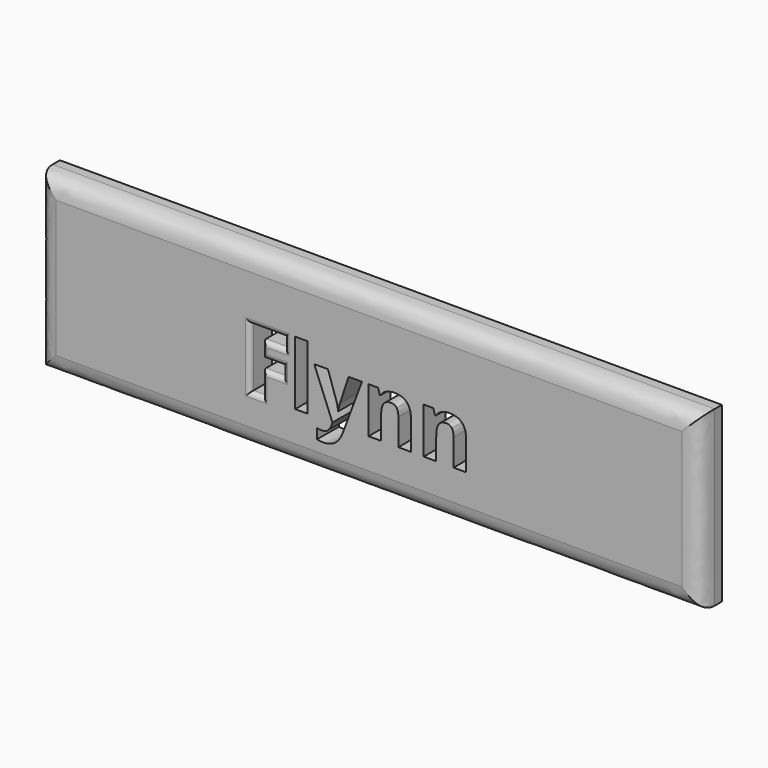
from build123d import *

# Parameters (mm, degrees)
F0_W        = 72.5492089987
F0_H        = 18.9791209996
F0_W_2      = 1.3700789067
F0_H_2      = 6.9912840748
F1_DEPTH    = 3
F2_T1_DEPTH = 82.5492089987
F2_T3_DEPTH = 28.9791209996
F3_R        = 0.5


# Not quite as in the source:
# - a fillet or chamfer that OpenCascade refuses, or shapes differently, is made with other operations: its cross-section is extruded or revolved along the edge and cut away or added


with BuildPart() as f1:
    # F0 (on Front) → F1 (new body)
    with BuildSketch(Plane.XZ):
        with Locations((-36.2746044993, 9.4895604998)):
            Rectangle(F0_W, F0_H)
        with BuildLine():
            Line((-40.2793404323, 5.3929338044), (-42.2747963845, 10.3801360367))
            Line((-42.2747963845, 10.3801360367), (-40.7738914752, 10.3801360367))
            Line((-40.7738914752, 10.3801360367), (-39.8264811924, 7.5537193204))
            add(Edge.make_bspline(
                [(-39.8264811924, 7.5537193204), (-39.70428108, 7.185681335), (-39.6597139803, 6.6825044018)],
                knots=[0, 0, 0, 1, 1, 1], degree=2))
            Line((-39.6597139803, 6.6825044018), (-39.632398661, 6.6825044018))
            add(Edge.make_bspline(
                [(-39.632398661, 6.6825044018), (-39.5835186161, 7.1454271804), (-39.439753778, 7.5537193204)],
                knots=[0, 0, 0, 1, 1, 1], degree=2))
            Line((-39.439753778, 7.5537193204), (-38.5095952758, 10.3801360367))
            Line((-38.5095952758, 10.3801360367), (-37.0403186308, 10.3801360367))
            Line((-37.0403186308, 10.3801360367), (-39.1651629373, 4.7143637688))
            add(Edge.make_bspline(
                [(-39.1651629373, 4.7143637688), (-39.458443207, 3.9279701046), (-39.9997178223, 3.5369297451)],
                knots=[0, 0, 0, 1, 1, 1], degree=2))
            add(Edge.make_bspline(
                [(-39.9997178223, 3.5369297451), (-40.5409924376, 3.1458893856), (-41.264129573, 3.1458893856)],
                knots=[0, 0, 0, 1, 1, 1], degree=2))
            add(Edge.make_bspline(
                [(-41.264129573, 3.1458893856), (-41.619228723, 3.1458893856), (-41.9599513892, 3.2235223981)],
                knots=[0, 0, 0, 1, 1, 1], degree=2))
            Line((-41.9599513892, 3.2235223981), (-41.9599513892, 4.3103845738))
            add(Edge.make_bspline(
                [(-41.9599513892, 4.3103845738), (-41.7126758677, 4.2514409902), (-41.4208332465, 4.2514409902)],
                knots=[0, 0, 0, 1, 1, 1], degree=2))
            add(Edge.make_bspline(
                [(-41.4208332465, 4.2514409902), (-41.0571082062, 4.2514409902), (-40.7853926623, 4.4742764892)],
                knots=[0, 0, 0, 1, 1, 1], degree=2))
            add(Edge.make_bspline(
                [(-40.7853926623, 4.4742764892), (-40.5136771183, 4.6971119882), (-40.36128639, 5.145658283)],
                knots=[0, 0, 0, 1, 1, 1], degree=2))
            Line((-40.36128639, 5.145658283), (-40.2793404323, 5.3929338044))
        make_face(mode=Mode.SUBTRACT)
        Polygon((-47.9362557073, 7.9533855702), (-47.9362557073, 5.3569925949), (-49.306334614, 5.3569925949), (-49.306334614, 11.9256080458), (-45.5411335052, 11.9256080458), (-45.5411335052, 10.7841152316), (-47.9362557073, 10.7841152316), (-47.9362557073, 9.0905654393), (-45.7079007174, 9.0905654393), (-45.7079007174, 7.9533855702), align=None, mode=Mode.SUBTRACT)
        with Locations((-43.6786600282, 8.8526346323)):
            Rectangle(F0_W_2, F0_H_2, mode=Mode.SUBTRACT)
        with BuildLine():
            Line((-31.6850784131, 8.6319556059), (-31.6850784131, 5.3569925949))
            Line((-31.6850784131, 5.3569925949), (-33.0551573198, 5.3569925949))
            Line((-33.0551573198, 5.3569925949), (-33.0551573198, 8.2912329397))
            add(Edge.make_bspline(
                [(-33.0551573198, 8.2912329397), (-33.0551573198, 8.8346640275), (-33.248521027, 9.1063795715)],
                knots=[0, 0, 0, 1, 1, 1], degree=2))
            add(Edge.make_bspline(
                [(-33.248521027, 9.1063795715), (-33.4418847342, 9.3780951154), (-33.8645533581, 9.3780951154)],
                knots=[0, 0, 0, 1, 1, 1], degree=2))
            add(Edge.make_bspline(
                [(-33.8645533581, 9.3780951154), (-34.4396127103, 9.3780951154), (-34.6955141221, 8.9942429978)],
                knots=[0, 0, 0, 1, 1, 1], degree=2))
            add(Edge.make_bspline(
                [(-34.6955141221, 8.9942429978), (-34.9514155338, 8.6103908802), (-34.9514155338, 7.7204865326)],
                knots=[0, 0, 0, 1, 1, 1], degree=2))
            Line((-34.9514155338, 7.7204865326), (-34.9514155338, 5.3569925949))
            Line((-34.9514155338, 5.3569925949), (-36.3214944405, 5.3569925949))
            Line((-36.3214944405, 5.3569925949), (-36.3214944405, 10.3801360367))
            Line((-36.3214944405, 10.3801360367), (-35.2748864195, 10.3801360367))
            Line((-35.2748864195, 10.3801360367), (-35.0908674267, 9.7375072106))
            Line((-35.0908674267, 9.7375072106), (-35.0146720626, 9.7375072106))
            add(Edge.make_bspline(
                [(-35.0146720626, 9.7375072106), (-34.7846483217, 10.1012322508), (-34.3828255993, 10.2874077161)],
                knots=[0, 0, 0, 1, 1, 1], degree=2))
            add(Edge.make_bspline(
                [(-34.3828255993, 10.2874077161), (-33.9810028769, 10.4735831814), (-33.4692000534, 10.4735831814)],
                knots=[0, 0, 0, 1, 1, 1], degree=2))
            add(Edge.make_bspline(
                [(-33.4692000534, 10.4735831814), (-32.5922345413, 10.4735831814), (-32.1386564772, 9.99987804)],
                knots=[0, 0, 0, 1, 1, 1], degree=2))
            add(Edge.make_bspline(
                [(-32.1386564772, 9.99987804), (-31.6850784131, 9.5261728986), (-31.6850784131, 8.6319556059)],
                knots=[0, 0, 0, 1, 1, 1], degree=2))
        make_face(mode=Mode.SUBTRACT)
        with BuildLine():
            Line((-25.6383293244, 8.6319556059), (-25.6383293244, 5.3569925949))
            Line((-25.6383293244, 5.3569925949), (-27.0084082311, 5.3569925949))
            Line((-27.0084082311, 5.3569925949), (-27.0084082311, 8.2912329397))
            add(Edge.make_bspline(
                [(-27.0084082311, 8.2912329397), (-27.0084082311, 8.8346640275), (-27.2017719383, 9.1063795715)],
                knots=[0, 0, 0, 1, 1, 1], degree=2))
            add(Edge.make_bspline(
                [(-27.2017719383, 9.1063795715), (-27.3951356454, 9.3780951154), (-27.8178042693, 9.3780951154)],
                knots=[0, 0, 0, 1, 1, 1], degree=2))
            add(Edge.make_bspline(
                [(-27.8178042693, 9.3780951154), (-28.3928636216, 9.3780951154), (-28.6487650333, 8.9942429978)],
                knots=[0, 0, 0, 1, 1, 1], degree=2))
            add(Edge.make_bspline(
                [(-28.6487650333, 8.9942429978), (-28.9046664451, 8.6103908802), (-28.9046664451, 7.7204865326)],
                knots=[0, 0, 0, 1, 1, 1], degree=2))
            Line((-28.9046664451, 7.7204865326), (-28.9046664451, 5.3569925949))
            Line((-28.9046664451, 5.3569925949), (-30.2747453518, 5.3569925949))
            Line((-30.2747453518, 5.3569925949), (-30.2747453518, 10.3801360367))
            Line((-30.2747453518, 10.3801360367), (-29.2281373307, 10.3801360367))
            Line((-29.2281373307, 10.3801360367), (-29.044118338, 9.7375072106))
            Line((-29.044118338, 9.7375072106), (-28.9679229738, 9.7375072106))
            add(Edge.make_bspline(
                [(-28.9679229738, 9.7375072106), (-28.7378992329, 10.1012322508), (-28.3360765105, 10.2874077161)],
                knots=[0, 0, 0, 1, 1, 1], degree=2))
            add(Edge.make_bspline(
                [(-28.3360765105, 10.2874077161), (-27.9342537882, 10.4735831814), (-27.4224509647, 10.4735831814)],
                knots=[0, 0, 0, 1, 1, 1], degree=2))
            add(Edge.make_bspline(
                [(-27.4224509647, 10.4735831814), (-26.5454854525, 10.4735831814), (-26.0919073884, 9.99987804)],
                knots=[0, 0, 0, 1, 1, 1], degree=2))
            add(Edge.make_bspline(
                [(-26.0919073884, 9.99987804), (-25.6383293244, 9.5261728986), (-25.6383293244, 8.6319556059)],
                knots=[0, 0, 0, 1, 1, 1], degree=2))
        make_face(mode=Mode.SUBTRACT)
    extrude(amount=F1_DEPTH)

    # F2: fillet of radius 2 on 4 edges, made by hand

    # F2_s2 → F2_t1 (cut)
    with BuildSketch(Plane.YZ.offset(-77.5492089987)):
        with BuildLine():
            add(Edge.make_bspline(
                [(-1, 18.9791209996), (-3, 18.9791209996), (-3, 16.9791209996)],
                knots=[0, 0, 0, 1, 1, 1], degree=2, weights=[1, 1, 1]))
            Line((-3, 16.9791209996), (-3, 18.9791209996))
            Line((-3, 18.9791209996), (-1, 18.9791209996))
        make_face()
        with BuildLine():
            add(Edge.make_bspline(
                [(-1, 0), (-3, 0), (-3, 2)],
                knots=[0, 0, 0, 1, 1, 1], degree=2, weights=[1, 1, 1]))
            Line((-3, 2), (-3, 0))
            Line((-3, 0), (-1, 0))
        make_face()
    extrude(amount=F2_T1_DEPTH, mode=Mode.SUBTRACT)

    # F2_s4 → F2_t3 (cut)
    with BuildSketch(Plane.XY.offset(-5)):
        with BuildLine():
            add(Edge.make_bspline(
                [(-72.5492089987, -1), (-72.5492089987, -3), (-70.5492089987, -3)],
                knots=[0, 0, 0, 1, 1, 1], degree=2, weights=[1, 1, 1]))
            Line((-70.5492089987, -3), (-72.5492089987, -3))
            Line((-72.5492089987, -3), (-72.5492089987, -1))
        make_face()
        with BuildLine():
            add(Edge.make_bspline(
                [(0, -1), (0, -3), (-2, -3)],
                knots=[0, 0, 0, 1, 1, 1], degree=2, weights=[1, 1, 1]))
            Line((-2, -3), (0, -3))
            Line((0, -3), (0, -1))
        make_face()
    extrude(amount=F2_T3_DEPTH, mode=Mode.SUBTRACT)

    # F3
    f3_edges = [f1.edges().sort_by_distance(p)[0] for p in [
        (-49.306335, -3, 8.6413),
        (-47.423734, -3, 11.925608),
        (-45.541134, -3, 11.354862),
        (-46.738695, -3, 10.784115),
        (-47.936256, -3, 9.93734),
        (-46.822078, -3, 9.090565),
        (-45.707901, -3, 8.521976),
        (-46.822078, -3, 7.953386),
        (-47.936256, -3, 6.655189),
        (-48.621295, -3, 5.356993),
    ]]
    fillet(f3_edges, radius=F3_R)


solid = f1.part
